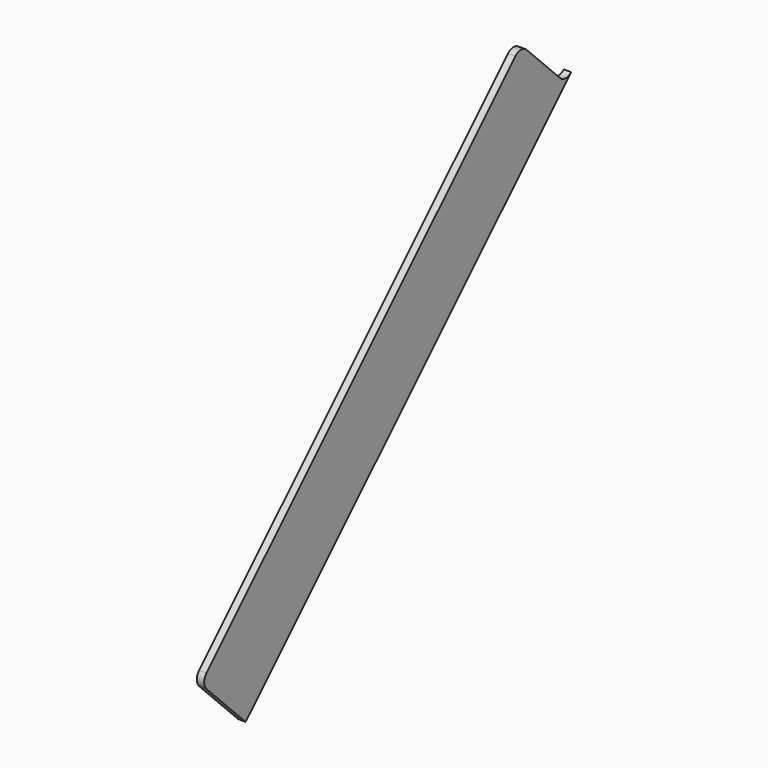
from build123d import *

# Parameters (mm, degrees)
F1_DEPTH = 4.7625


# Not quite as in the source:
# - ends of sketch curves that miss each other by under 0.0002 mm in the source are joined


with BuildPart() as f1:
    # F0 (on Right) → F1 (new body)
    with BuildSketch(Plane.YZ):
        with BuildLine():
            ThreePointArc((-10.3035716562, 255.2451451351), (-14.739191866, 253.5576398603), (-19.1058595605, 255.4162990395))
            Line((-19.1058595605, 255.4162990395), (-19.2069466, 255.517396))
            Line((-19.2069466, 255.517396), (-46.1477106, 282.45816))
            ThreePointArc((-46.1477106, 282.45816), (-50.6378374197, 284.3180242), (-55.1279617605, 282.4581649605))
            Line((-55.1279617605, 282.4581649605), (-303.1270036, 34.4591132))
            ThreePointArc((-303.1270036, 34.4591132), (-304.9868678, 29.9689938197), (-303.1269958605, 25.4788747395))
            Line((-303.1269958605, 25.4788747395), (-271.6961038, -5.9520328))
            Line((-271.6961038, -5.9520328), (-10.3035716562, 255.2451451351))
        make_face()
    extrude(amount=F1_DEPTH)


solid = f1.part
